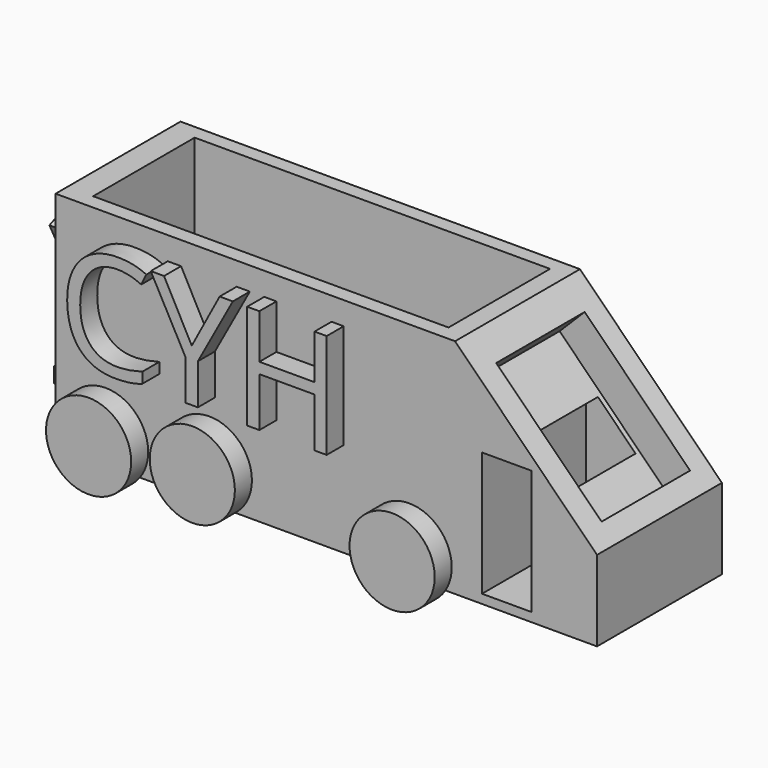
from build123d import *

# Parameters (mm, degrees)
F0_W          = 193.7721520662
F0_H          = 79.6380527318
F1_DEPTH      = 55.88
F2_SIZE       = 50.8
F3_W          = 17.78
F3_H          = 44.5166216948
F4_DEPTH      = 46.482
F5_W          = 39.5805523731
F5_H          = 53.3422920853
F6_DEPTH      = 12.7
F7_W          = 127.1854564548
F7_H          = 45.4278131947
F8_DEPTH      = 67.056
F9_R          = 15.24
F10_DEPTH     = 7.62
F11_R         = 15.24
F12_DEPTH     = 7.62
F13_R         = 15.24
F14_DEPTH     = 7.62
F15_R         = 15.24
F16_DEPTH     = 7.62
F17_TEXT_SIZE = 47.4981756674
F18_DEPTH     = 7.62
F19_TEXT_SIZE = 52.4653070089
F20_DEPTH     = 7.62
F21_TEXT_SIZE = 76.283435007
F22_DEPTH     = 7.62
F23_W         = 58.9049998671
F23_H         = 17.3249989748
F24_DEPTH     = 3.81
F25_W         = 5.2607059479
F25_H         = 10.7412729412
F25_W_2       = 9.150584694
F25_H_2       = 14.8033723235
F25_W_3       = 4.7578979284
F25_H_3       = 20.6869645044
F25_W_4       = 12.3569229618
F25_H_4       = 19.3955469877
F25_W_5       = 9.4247497618
F25_H_5       = 16.1392129958
F25_W_6       = 7.3692561127
F25_H_6       = 11.7015270516
F25_W_7       = 8.3871111274
F25_H_7       = 12.8826694563
F25_W_8       = 2.3494400084
F25_H_8       = 10.3444037959
F25_W_9       = 7.7797686681
F25_H_9       = 8.1241950393
F25_W_10      = 11.6106481291
F25_H_10      = 11.5989008918
F25_W_11      = 4.9952003174
F25_H_11      = 9.3175470829
F25_W_12      = 3.1682215631
F25_H_12      = 6.6125765443
F26_DEPTH     = 25.4


# Not quite as in the source:
# - Text() gives the source's letters only with a copy of the font that has no kerning and outlines rounded to 1/6400 em; it was checked with that copy


with BuildPart() as f1:
    # F0 (on Front) → F1 (new body)
    with BuildSketch(Plane.XZ):
        with Locations((24.3605226278, 5.8698412031)):
            Rectangle(F0_W, F0_H)
    extrude(amount=F1_DEPTH)

    # F2
    f2_edges = [f1.edges().sort_by_distance(p)[0] for p in [
        (121.246599, -27.94, 45.688868),
    ]]
    chamfer(f2_edges, length=F2_SIZE)

    # F3 (on face) → F4 (cut)
    with BuildSketch(Plane.XZ.offset(55.88)):
        with Locations((88.9713466167, -8.4744174965)):
            Rectangle(F3_W, F3_H)
    extrude(amount=-F4_DEPTH, mode=Mode.SUBTRACT)

    # F5 (on face) → F6 (cut)
    with BuildSketch(Plane(origin=(58.067733115, 0, 58.067733115), x_dir=(0, 1, 0), z_dir=(0.7071067812, 0, 0.7071067812))):
        with Locations((-27.4632207584, -55.2427796647)):
            Rectangle(F5_W, F5_H)
    extrude(amount=-F6_DEPTH, mode=Mode.SUBTRACT)

    # F7 (on face) → F8 (cut)
    with BuildSketch(Plane.XY.offset(45.688867569)):
        with Locations((0.2324543893, -27.822334785)):
            Rectangle(F7_W, F7_H)
    extrude(amount=-F8_DEPTH, mode=Mode.SUBTRACT)

    # F9 (on face) → F10 (join)
    with BuildSketch(Plane.XZ.offset(55.88)):
        with Locations((-54.6228326857, -24.9125752598)):
            Circle(F9_R)
        with Locations((54.0145672858, -25.9398017079)):
            Circle(F9_R)
    extrude(amount=F10_DEPTH)

    # F11 (on face) → F12 (join)
    with BuildSketch(Plane(origin=(0, 0, 0), x_dir=(-1, 0, 0), z_dir=(0, 1, 0))):
        with Locations((56.5575473011, -25.3813583404)):
            Circle(F11_R)
        with Locations((-53.8387522101, -23.8742418587)):
            Circle(F11_R)
    extrude(amount=F12_DEPTH)

    # F13 (on face) → F14 (join)
    with BuildSketch(Plane(origin=(0, 0, 0), x_dir=(-1, 0, 0), z_dir=(0, 1, 0))):
        with Locations((18.8156589866, -24.9382779002)):
            Circle(F13_R)
    extrude(amount=F14_DEPTH)

    # F15 (on face) → F16 (join)
    with BuildSketch(Plane.XZ.offset(55.88)):
        with Locations((-17.5050161779, -21.820710972)):
            Circle(F15_R)
    extrude(amount=F16_DEPTH)

    # F17 (on face) → F18 (join)
    with BuildSketch(Plane(origin=(0, 0, 0), x_dir=(-1, 0, 0), z_dir=(0, 1, 0))):
        with Locations((-68.0814161897, 0)):
            Text('CYH', F17_TEXT_SIZE, font='Open Sans', text_align=(TextAlign.LEFT, TextAlign.BOTTOM))
    extrude(amount=F18_DEPTH)

    # F19 (on face) → F20 (join)
    with BuildSketch(Plane.XZ.offset(55.88)):
        with Locations((-65.4820874333, 0)):
            Text('CYH', F19_TEXT_SIZE, font='Open Sans', text_align=(TextAlign.LEFT, TextAlign.BOTTOM))
    extrude(amount=F20_DEPTH)

    # F21 (on face) → F22 (join)
    with BuildSketch(Plane(origin=(-72.5255534053, 0, 0), x_dir=(0, -1, 0), z_dir=(-1, 0, 0))):
        with Locations((3.2569264527, -21.6046524902)):
            Text('C', F21_TEXT_SIZE, font='Open Sans', text_align=(TextAlign.LEFT, TextAlign.BOTTOM))
    extrude(amount=F22_DEPTH)

    # F23 (on face) → F24 (join)
    with BuildSketch(Plane(origin=(0, 0, -33.9491851628), x_dir=(1, 0, 0), z_dir=(0, 0, -1))):
        with Locations((-12.0519762859, 32.2875007987)):
            Rectangle(F23_W, F23_H)
    extrude(amount=F24_DEPTH)

    # F25 (on face) → F26 (join)
    with BuildSketch(Plane.XY.offset(-21.367132431)):
        with Locations((27.5665484369, -35.1522443816)):
            Rectangle(F25_W, F25_H)
        with Locations((9.4830405433, -31.7002013326)):
            Rectangle(F25_W_2, F25_H_2)
        with Locations((25.7008643821, -15.4519104399)):
            Rectangle(F25_W_3, F25_H_3)
        with Locations((-18.6509522609, -31.3966749236)):
            Rectangle(F25_W_4, F25_H_4)
        with Locations((-44.2849267274, -29.4862743467)):
            Rectangle(F25_W_5, F25_H_5)
        with Locations((-3.6846280564, -14.45225114)):
            Rectangle(F25_W_6, F25_H_6)
        with Locations((-37.9337929189, -11.5497629158)):
            Rectangle(F25_W_7, F25_H_7)
        with Locations((-55.2138704807, -13.7392976321)):
            Rectangle(F25_W_8, F25_H_8)
        with Locations((-18.9724867232, -12.7329174429)):
            Rectangle(F25_W_9, F25_H_9)
        with Locations((9.8069540691, -14.4009380601)):
            Rectangle(F25_W_10, F25_H_10)
        with Locations((-2.4976001587, -34.2034585774)):
            Rectangle(F25_W_11, F25_H_11)
        with Locations((-32.0725012571, -32.7352397144)):
            Rectangle(F25_W_12, F25_H_12)
    extrude(amount=F26_DEPTH)


solid = f1.part
